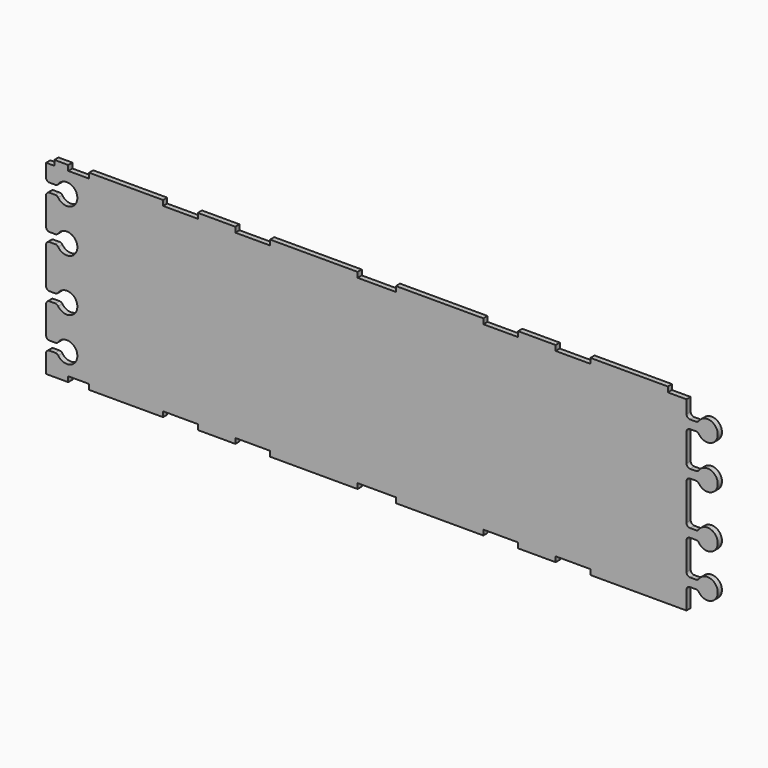
from build123d import *

# Parameters (mm, degrees)
F0_W     = 16.768251
F0_H     = 110
F0_W_2   = 16.76825
F1_DEPTH = 3


# Not quite as in the source:
# - ends of sketch curves that miss each other by under 0.0002 mm in the source are joined


with BuildPart() as f1:
    # F0 (on Front) → F1 (new body)
    with BuildSketch(Plane.XZ):
        with BuildLine():
            Line((-165.473004, -55), (-165.473004, 55))
            Line((-165.473004, 55), (-168.473004, 55))
            Line((-168.473004, 55), (-168.473004, 52))
            Line((-168.473004, 52), (-180.473004, 52))
            Line((-180.473004, 52), (-180.473004, 55))
            Line((-180.473004, 55), (-188.473004, 55))
            Line((-188.473004, 55), (-188.473004, 52))
            Line((-188.473004, 52), (-193.223004, 52))
            Line((-193.223004, 52), (-193.223004, 44.5))
            ThreePointArc((-193.223004, 44.5), (-192.6518622233, 43.1211417767), (-191.273004, 42.55))
            Line((-191.273004, 42.55), (-187.887382, 42.55))
            ThreePointArc((-187.887382, 42.55), (-186.9753529387, 42.7764272596), (-186.2751272015, 43.4031251371))
            ThreePointArc((-186.2751272015, 43.4031251371), (-175.223004, 40), (-186.2751273913, 36.5968747338))
            ThreePointArc((-186.2751273913, 36.5968747338), (-186.9753529387, 37.2235727404), (-187.887382, 37.45))
            Line((-187.887382, 37.45), (-191.273004, 37.45))
            ThreePointArc((-191.273004, 37.45), (-192.6518622233, 36.8788582233), (-193.223004, 35.5))
            Line((-193.223004, 35.5), (-193.223004, 19.5))
            ThreePointArc((-193.223004, 19.5), (-192.6518622233, 18.1211417767), (-191.273004, 17.55))
            Line((-191.273004, 17.55), (-187.887382, 17.55))
            ThreePointArc((-187.887382, 17.55), (-186.9753529387, 17.7764272596), (-186.2751272015, 18.4031251371))
            ThreePointArc((-186.2751272015, 18.4031251371), (-175.223004, 15), (-186.2751273913, 11.5968747338))
            ThreePointArc((-186.2751273913, 11.5968747338), (-186.9753529387, 12.2235727404), (-187.887382, 12.45))
            Line((-187.887382, 12.45), (-191.273004, 12.45))
            ThreePointArc((-191.273004, 12.45), (-192.6518622233, 11.8788582233), (-193.223004, 10.5))
            Line((-193.223004, 10.5), (-193.223004, -10.5))
            ThreePointArc((-193.223004, -10.5), (-192.6518622233, -11.8788582233), (-191.273004, -12.45))
            Line((-191.273004, -12.45), (-187.887382, -12.45))
            ThreePointArc((-187.887382, -12.45), (-186.9753529387, -12.2235727404), (-186.2751272015, -11.5968748629))
            ThreePointArc((-186.2751272015, -11.5968748629), (-175.223004, -15), (-186.2751273913, -18.4031252662))
            ThreePointArc((-186.2751273913, -18.4031252662), (-186.9753529387, -17.7764272596), (-187.887382, -17.55))
            Line((-187.887382, -17.55), (-191.273004, -17.55))
            ThreePointArc((-191.273004, -17.55), (-192.6518622233, -18.1211417767), (-193.223004, -19.5))
            Line((-193.223004, -19.5), (-193.223004, -35.5))
            ThreePointArc((-193.223004, -35.5), (-192.6518622233, -36.8788582233), (-191.273004, -37.45))
            Line((-191.273004, -37.45), (-187.887382, -37.45))
            ThreePointArc((-187.887382, -37.45), (-186.9753529387, -37.2235727404), (-186.2751272015, -36.5968748629))
            ThreePointArc((-186.2751272015, -36.5968748629), (-175.223004, -40), (-186.2751273913, -43.4031252662))
            ThreePointArc((-186.2751273913, -43.4031252662), (-186.9753529387, -42.7764272596), (-187.887382, -42.55))
            Line((-187.887382, -42.55), (-191.273004, -42.55))
            ThreePointArc((-191.273004, -42.55), (-192.6518622233, -43.1211417767), (-193.223004, -44.5))
            Line((-193.223004, -44.5), (-193.223004, -55))
            Line((-193.223004, -55), (-180.473004, -55))
            Line((-180.473004, -55), (-180.473004, -52))
            Line((-180.473004, -52), (-168.473004, -52))
            Line((-168.473004, -52), (-168.473004, -55))
            Line((-168.473004, -55), (-165.473004, -55))
        make_face()
        with Locations((-157.0888785, 0)):
            Rectangle(F0_W, F0_H)
        with Locations((-140.3206275, 0)):
            Rectangle(F0_W, F0_H)
        Polygon((-58.336502, -55), (-58.336502, 55), (-64.336502, 55), (-64.336502, 52), (-84.336502, 52), (-84.336502, 55), (-105.936502, 55), (-105.936502, 52), (-125.936502, 52), (-125.936502, 55), (-131.936502, 55), (-131.936502, -55), (-125.936502, -55), (-125.936502, -52), (-105.936502, -52), (-105.936502, -55), (-84.336502, -55), (-84.336502, -52), (-64.336502, -52), (-64.336502, -55), align=None)
        with Locations((-33.1841255, 0)):
            Rectangle(F0_W, F0_H)
        Polygon((18.8, -55), (18.8, 55), (8, 55), (8, 52), (-14, 52), (-14, 55), (-24.8, 55), (-24.8, -55), (-14, -55), (-14, -52), (8, -52), (8, -55), align=None)
        with Locations((27.184125, 0)):
            Rectangle(F0_W_2, F0_H)
        with Locations((43.9523755, 0)):
            Rectangle(F0_W, F0_H)
        Polygon((125.936501, -55), (125.936501, 55), (119.936501, 55), (119.936501, 52), (99.936501, 52), (99.936501, 55), (78.336501, 55), (78.336501, 52), (58.336501, 52), (58.336501, 55), (52.336501, 55), (52.336501, -55), (58.336501, -55), (58.336501, -52), (78.336501, -52), (78.336501, -55), (99.936501, -55), (99.936501, -52), (119.936501, -52), (119.936501, -55), align=None)
        with Locations((134.3206265, 0)):
            Rectangle(F0_W, F0_H)
        with Locations((151.0888775, 0)):
            Rectangle(F0_W, F0_H)
        with BuildLine():
            Line((164.473003, 55), (159.473003, 55))
            Line((159.473003, 55), (159.473003, -55))
            Line((159.473003, -55), (175.223003, -55))
            Line((175.223003, -55), (175.223003, -44.5))
            ThreePointArc((175.223003, -44.5), (175.8234340986, -43.0504310986), (177.273003, -42.45))
            Line((177.273003, -42.45), (180.658624, -42.45))
            ThreePointArc((180.658624, -42.45), (181.6174238462, -42.6880389477), (182.3535586128, -43.3468752634))
            ThreePointArc((182.3535586128, -43.3468752634), (193.223003, -40), (182.3535591066, -36.6531250725))
            ThreePointArc((182.3535591066, -36.6531250725), (181.6174238462, -37.3119610523), (180.658624, -37.55))
            Line((180.658624, -37.55), (177.273003, -37.55))
            ThreePointArc((177.273003, -37.55), (175.8234340986, -36.9495689014), (175.223003, -35.5))
            Line((175.223003, -35.5), (175.223003, -19.5))
            ThreePointArc((175.223003, -19.5), (175.8234340986, -18.0504310986), (177.273003, -17.45))
            Line((177.273003, -17.45), (180.658624, -17.45))
            ThreePointArc((180.658624, -17.45), (181.6174238462, -17.6880389477), (182.3535586128, -18.3468752634))
            ThreePointArc((182.3535586128, -18.3468752634), (193.223003, -15), (182.3535591066, -11.6531250725))
            ThreePointArc((182.3535591066, -11.6531250725), (181.6174238462, -12.3119610523), (180.658624, -12.55))
            Line((180.658624, -12.55), (177.273003, -12.55))
            ThreePointArc((177.273003, -12.55), (175.8234340986, -11.9495689014), (175.223003, -10.5))
            Line((175.223003, -10.5), (175.223003, 10.5))
            ThreePointArc((175.223003, 10.5), (175.8234340986, 11.9495689014), (177.273003, 12.55))
            Line((177.273003, 12.55), (180.658624, 12.55))
            ThreePointArc((180.658624, 12.55), (181.6174238462, 12.3119610523), (182.3535586128, 11.6531247366))
            ThreePointArc((182.3535586128, 11.6531247366), (193.223003, 15), (182.3535591066, 18.3468749275))
            ThreePointArc((182.3535591066, 18.3468749275), (181.6174238462, 17.6880389477), (180.658624, 17.45))
            Line((180.658624, 17.45), (177.273003, 17.45))
            ThreePointArc((177.273003, 17.45), (175.8234340986, 18.0504310986), (175.223003, 19.5))
            Line((175.223003, 19.5), (175.223003, 35.5))
            ThreePointArc((175.223003, 35.5), (175.8234340986, 36.9495689014), (177.273003, 37.55))
            Line((177.273003, 37.55), (180.658624, 37.55))
            ThreePointArc((180.658624, 37.55), (181.6174238462, 37.3119610523), (182.3535586128, 36.6531247366))
            ThreePointArc((182.3535586128, 36.6531247366), (193.223003, 40), (182.3535591066, 43.3468749275))
            ThreePointArc((182.3535591066, 43.3468749275), (181.6174238462, 42.6880389477), (180.658624, 42.45))
            Line((180.658624, 42.45), (177.273003, 42.45))
            ThreePointArc((177.273003, 42.45), (175.8234340986, 43.0504310986), (175.223003, 44.5))
            Line((175.223003, 44.5), (175.223003, 52))
            Line((175.223003, 52), (164.473003, 52))
            Line((164.473003, 52), (164.473003, 55))
        make_face()
        with Locations((-49.9523765, 0)):
            Rectangle(F0_W, F0_H)
    extrude(amount=F1_DEPTH)


solid = f1.part
